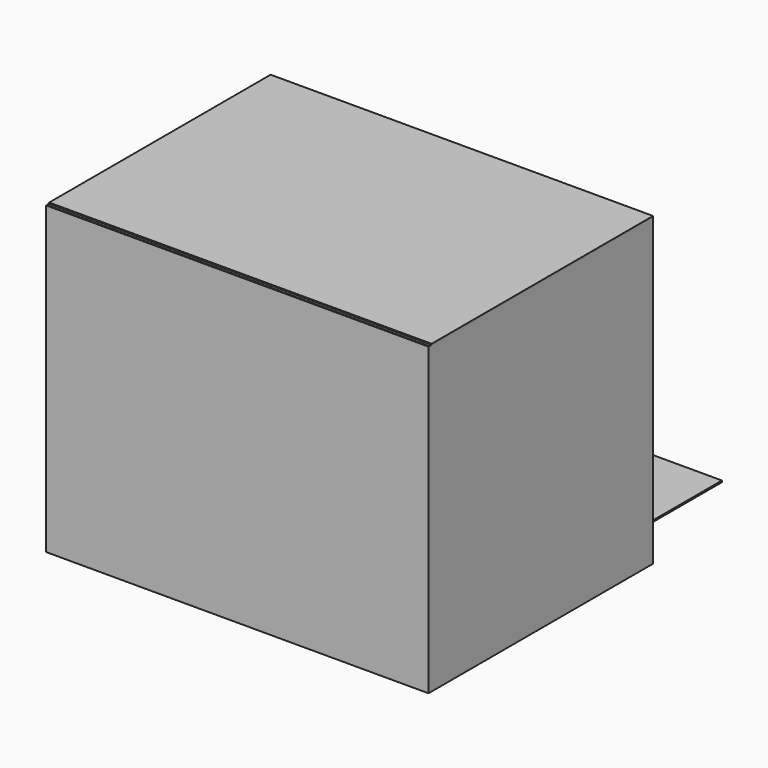
from build123d import *

# Parameters (mm, degrees)
F0_W      = 762
F0_H      = 558.8
F1_DEPTH  = 3.03784
F2_W      = 558.8
F2_H      = 609.6
F3_DEPTH  = 1.89738
F4_W      = 762
F4_H      = 609.6
F5_DEPTH  = 1.89738
F6_W      = 558.8
F6_H      = 609.6
F7_DEPTH  = 1.89738
F8_W      = 762
F8_H      = 601.345
F9_DEPTH  = 1.89738
F10_W     = 763.89738
F10_H     = 552.9529485043
F11_DEPTH = 1.89738


with BuildPart() as f1:
    # F0 (on Top) → F1 (new body)
    with BuildSketch(Plane.XY):
        Rectangle(F0_W, F0_H)
    extrude(amount=F1_DEPTH)


with BuildPart() as f3:
    # F2 (on face) → F3 (new body)
    with BuildSketch(Plane.YZ.offset(381)):
        with Locations((-174.2725175381, 232.979187201)):
            Rectangle(F2_W, F2_H)
    extrude(amount=F3_DEPTH)

    # F4 (on face) → F5 (join)
    with BuildSketch(Plane.XZ.offset(453.6725175381)):
        with Locations((1.89738, 232.979187201)):
            Rectangle(F4_W, F4_H)
    extrude(amount=F5_DEPTH)

    # F6 (on face) → F7 (join)
    with BuildSketch(Plane(origin=(-379.10262, 0, 0), x_dir=(0, -1, 0), z_dir=(-1, 0, 0))):
        with Locations((176.1698975381, 232.979187201)):
            Rectangle(F6_W, F6_H)
    extrude(amount=F7_DEPTH)

    # F8 (on face) → F9 (join)
    with BuildSketch(Plane(origin=(0, 103.2301024619, 0), x_dir=(-1, 0, 0), z_dir=(0, 1, 0))):
        with Locations((0, 228.851687201)):
            Rectangle(F8_W, F8_H)
    extrude(amount=F9_DEPTH)


with BuildPart() as f11:
    # F10 (on face) → F11 (new body)
    with BuildSketch(Plane.XY.offset(537.779187201)):
        with Locations((0.94869, -171.3489917902)):
            Rectangle(F10_W, F10_H)
    extrude(amount=F11_DEPTH)


solid = Compound([f1.part, f3.part, f11.part])
